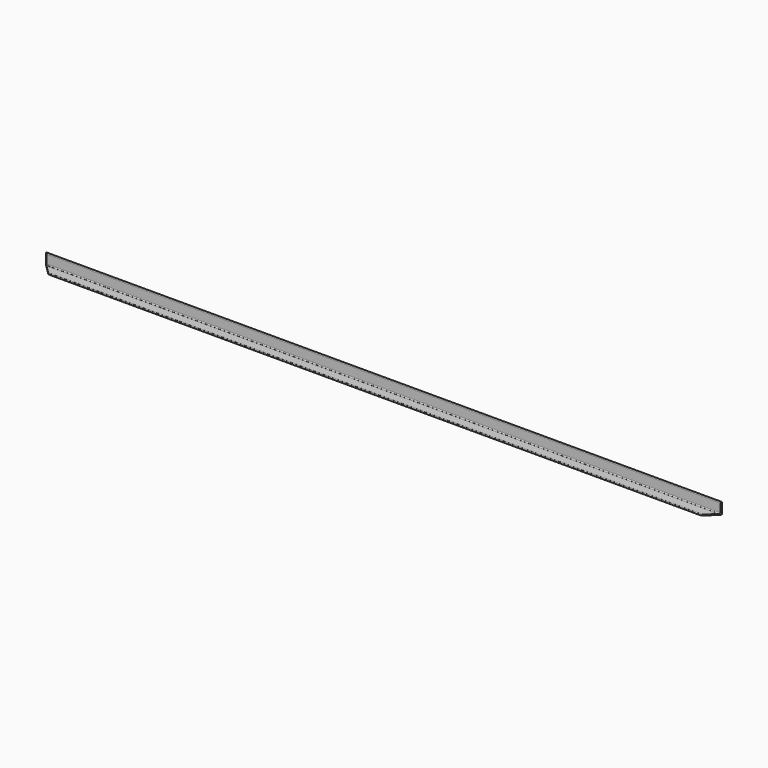
from build123d import *

# Parameters (mm, degrees)
F1_DEPTH = 1500
F3_DEPTH = 50.001


# Not quite as in the source:
# - a pattern or mirror of a feature is missing from the dataset's text; its kind, count and spacing are read off the source's solid


with BuildPart() as f1:
    # F0 (on Right) → F1 (new body, symmetric)
    with BuildSketch(Plane.YZ):
        with BuildLine():
            Line((0, 0), (0, 50))
            ThreePointArc((0, 50), (-2.8284271247, 48.8284271247), (-4, 46))
            Line((-4, 46), (-4, 8))
            ThreePointArc((-4, 8), (-5.1715728753, 5.1715728753), (-8, 4))
            Line((-8, 4), (-46, 4))
            ThreePointArc((-46, 4), (-48.8284271247, 2.8284271247), (-50, 0))
            Line((-50, 0), (0, 0))
        make_face()
    extrude(amount=F1_DEPTH, both=True)

    # F2 (on face) → F3 (cut, through all)
    with BuildSketch(Plane(origin=(0, 0, 0), x_dir=(1, 0, 0), z_dir=(0, 0, -1))):
        Polygon((1450, 50), (1500, 0), (1500, 50), align=None)
    f3 = extrude(amount=-F3_DEPTH, mode=Mode.SUBTRACT)

    # F3_copies: F3 across plane
    add(f3.mirror(Plane(origin=(0, 0, 0), x_dir=(0, 0, -1), z_dir=(-1, 0, 0))), mode=Mode.SUBTRACT)


solid = f1.part
